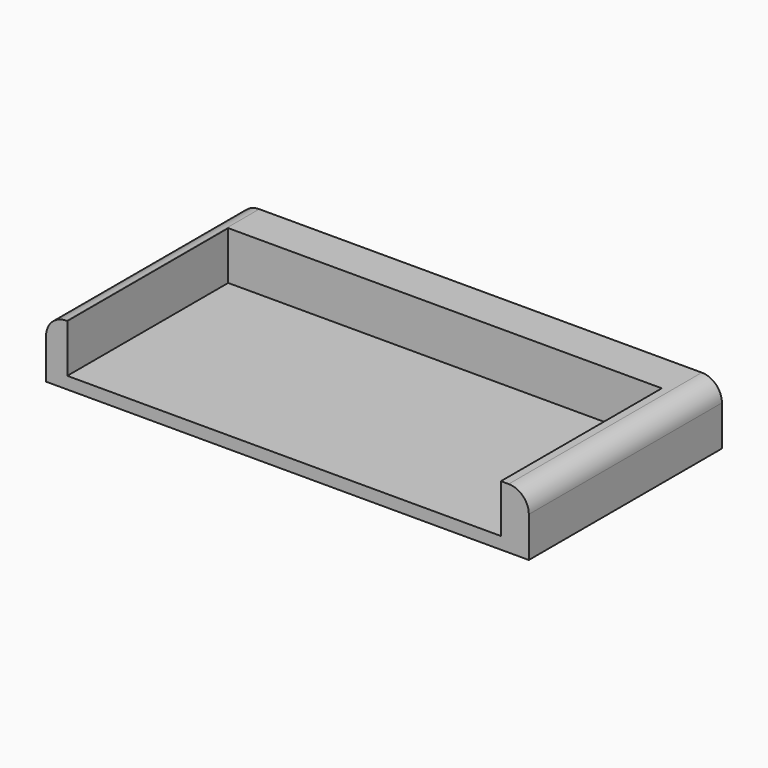
from build123d import *

# Parameters (mm, degrees)
F0_W     = 107.7930156246
F0_H     = 50
F1_DEPTH = 3
F2_DEPTH = 15
F3_R     = 5
F3_2_R   = 5
F5_W     = 52
F5_H     = 11
F6_DEPTH = 3


with BuildPart() as f1:
    # F0 (on Top) → F1 (new body)
    with BuildSketch(Plane.XY):
        Polygon((-57.7105433475, 0), (-57.7105433475, -50), (-52.4395332623, -50), (-52.4395332623, 0), (55.3534823623, 0), (55.3534823623, -50), (62.2894566525, -50), (62.2894566525, 0), (62.2894566525, 10), (-57.7105433475, 10), align=None)
        with Locations((1.45697455, -25)):
            Rectangle(F0_W, F0_H)
    extrude(amount=F1_DEPTH)

    # F3#2
    f3_2_edges = [f1.edges().sort_by_distance(p)[0] for p in [
        (-57.710543, -50, 1.5),
        (62.289457, -50, 1.5),
    ]]
    fillet(f3_2_edges, radius=F3_2_R)


with BuildPart() as f2:
    # F0 (on Top) → F2 (new body)
    with BuildSketch(Plane.XY):
        Polygon((-57.7105433475, 0), (-57.7105433475, -50), (-52.4395332623, -50), (-52.4395332623, 0), (55.3534823623, 0), (55.3534823623, -50), (62.2894566525, -50), (62.2894566525, 0), (62.2894566525, 10), (-57.7105433475, 10), align=None)
    extrude(amount=F2_DEPTH)

    # F3
    f3_edges = [f2.edges().sort_by_distance(p)[0] for p in [
        (-57.710543, -20, 15),
        (62.289457, -20, 15),
    ]]
    fillet(f3_edges, radius=F3_R)


with BuildPart() as f1_1:
    add(f1.part)

    # F4: union F2
    add(f2.part)

    # F5 (on face) → F6 (cut)
    with BuildSketch(Plane(origin=(0, 10, 0), x_dir=(-1, 0, 0), z_dir=(0, 1, 0))):
        with Locations((-1.9977902994, 7.5)):
            Rectangle(F5_W, F5_H)
    extrude(amount=-F6_DEPTH, mode=Mode.SUBTRACT)


solid = f1_1.part
